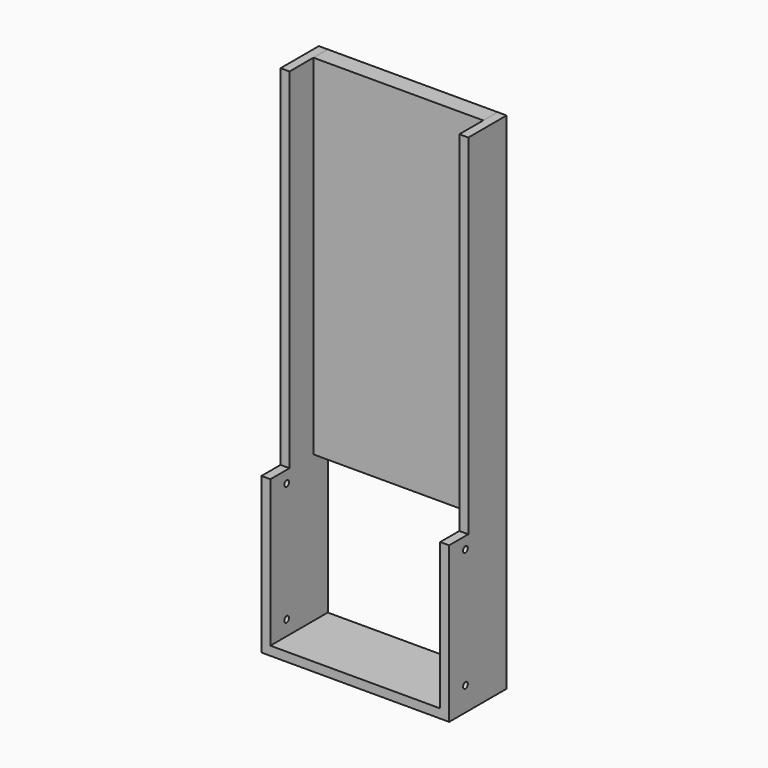
from build123d import *

# Parameters (mm, degrees)
F0_W     = 180.34
F0_H     = 370.84
F1_DEPTH = 19.05
F4_DEPTH = 9.525
F6_W     = 76.2
F6_H     = 9.525
F7_DEPTH = 180.34
F8_R     = 3.175
F9_DEPTH = 199.391


with BuildPart() as f1:
    # F0 (on Front) → F1 (new body)
    with BuildSketch(Plane.XZ):
        Rectangle(F0_W, F0_H)
    extrude(amount=F1_DEPTH)


with BuildPart() as f4:
    # F3 (on face) → F4 (new body)
    with BuildSketch(Plane(origin=(-90.17, 0, 0), x_dir=(0, -1, 0), z_dir=(-1, 0, 0))):
        Polygon((50.8, 185.42), (0, 185.42), (0, -350.52), (50.8, -350.52), (76.2, -350.52), (76.2, -185.42), (50.8, -185.42), align=None)
    extrude(amount=F4_DEPTH)


with BuildPart() as f5_1:
    # F5: instance of F4
    add(f4.part.mirror(Plane.YZ))


with BuildPart() as f4_1:
    add(f4.part)

    add(f5_1.part)  # F7 merges F5_1
    # F6 (on face) → F7 (join, through all)
    with BuildSketch(Plane(origin=(90.17, 0, 0), x_dir=(0, -1, 0), z_dir=(-1, 0, 0))):
        with Locations((38.1, -345.7575)):
            Rectangle(F6_W, F6_H)
    extrude(amount=F7_DEPTH)

    # F8 (on face) → F9 (cut, through all)
    with BuildSketch(Plane(origin=(-99.695, 0, 0), x_dir=(0, -1, 0), z_dir=(-1, 0, 0))):
        with Locations((54.61, -198.12)):
            Circle(F8_R)
        with Locations((54.61, -325.12)):
            Circle(F8_R)
    extrude(amount=-F9_DEPTH, mode=Mode.SUBTRACT)


solid = Compound([f1.part, f4_1.part])
